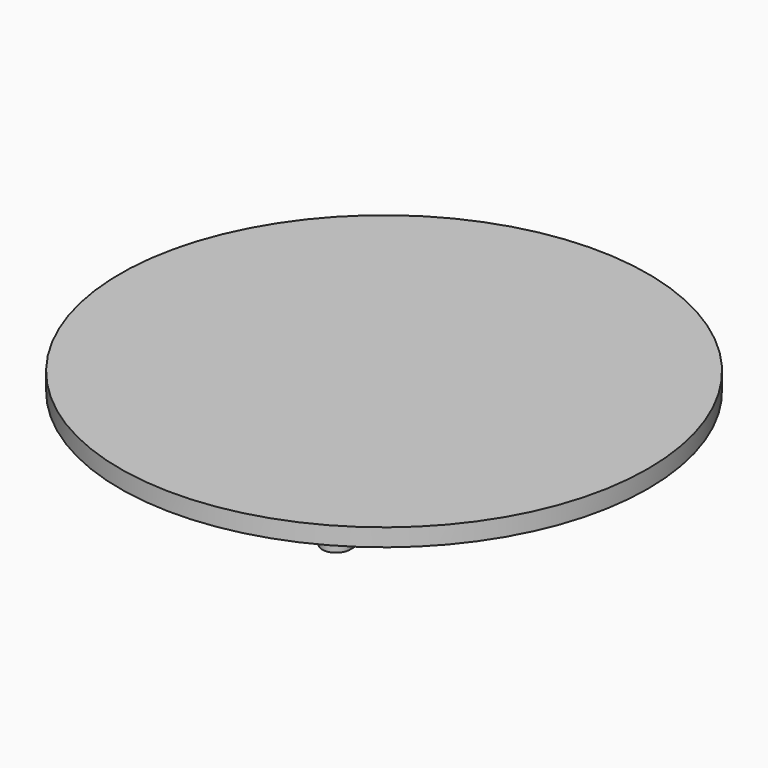
from build123d import *

# Parameters (mm, degrees)
F0_R            = 6.5
F1_DEPTH        = 11
F2_R            = 0.75
F3_DEPTH        = 6
F4_R            = 1
F5_DEPTH        = 1.5
F5_COPIES_COUNT = 3
F6_SIZE2        = 2.54
F6_SIZE         = 5.08
F7_R            = 38.1
F8_DEPTH        = 2.54


# Not quite as in the source:
# - a pattern or mirror of a feature is missing from the dataset's text; its kind, count and spacing are read off the source's solid


with BuildPart() as f1:
    # F0 (on Top) → F1 (new body)
    with BuildSketch(Plane.XY):
        Circle(F0_R)
    extrude(amount=F1_DEPTH)

    # F2 (on face) → F3 (join)
    with BuildSketch(Plane.XY.offset(11)):
        Circle(F2_R)
    extrude(amount=F3_DEPTH)

    # F4 (on face) → F5 (join)
    with BuildSketch(Plane(origin=(0, 0, 0), x_dir=(1, 0, 0), z_dir=(0, 0, -1))):
        with BuildLine():
            ThreePointArc((2, 8.6602540378), (0, 10.6602540378), (-2, 8.6602540378))
            Line((-2, 8.6602540378), (-2, 2.2360679775))
            ThreePointArc((-2, 2.2360679775), (-2.3283095216, 1.8918178485), (-2.5980762114, 1.5))
            Line((-2.5980762114, 1.5), (0, 0))
            Line((0, 0), (2.5980762114, 1.5))
            ThreePointArc((2.5980762114, 1.5), (2.3283095216, 1.8918178485), (2, 2.2360679775))
            Line((2, 2.2360679775), (2, 8.6602540378))
        make_face()
        with Locations((0, 8.6602540378)):
            Circle(F4_R, mode=Mode.SUBTRACT)
    f5 = extrude(amount=F5_DEPTH)

    # F5_copies: F5 ×3 about axis
    f5_copies_axis = Axis((0, 0, 0), (0, 0, 1))
    for i in range(1, F5_COPIES_COUNT):
        add(f5.rotate(f5_copies_axis, i * 360 / F5_COPIES_COUNT))

    # F6
    f6_edges = [f1.edges().sort_by_distance(p)[0] for p in [
        (-6.5, 0, 11),
    ]]
    f6_side = f1.faces().sort_by_distance((-6.316152, 0, 11))[0]
    chamfer(f6_edges, length=F6_SIZE, length2=F6_SIZE2, reference=f6_side)

    # F7 (on face) → F8 (join)
    with BuildSketch(Plane.XY.offset(17)):
        Circle(F7_R)
    extrude(amount=-F8_DEPTH)


solid = f1.part
